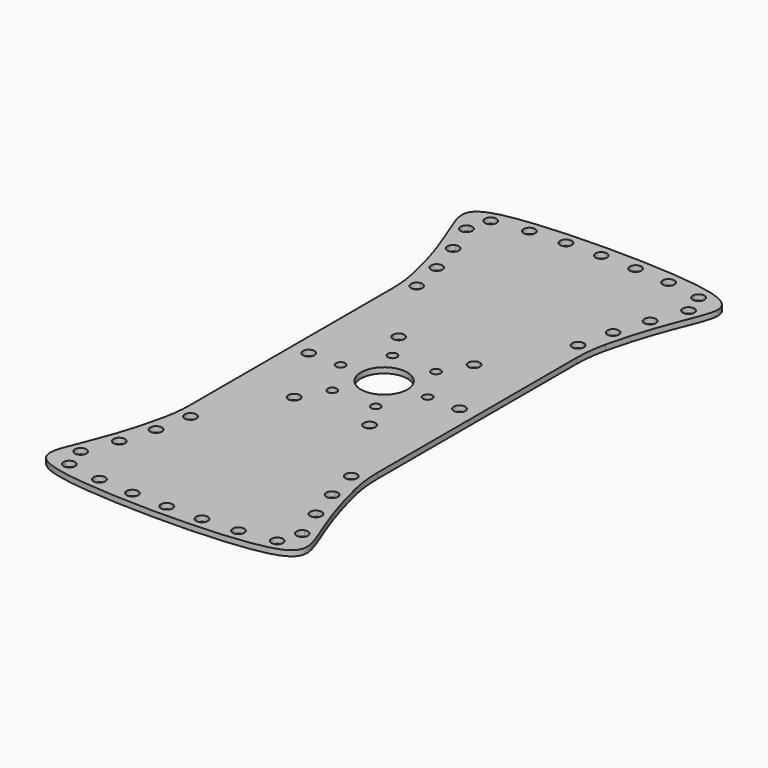
from build123d import *

# Parameters (mm, degrees)
F1_DEPTH = 2.9972
F2_R     = 2.54
F2_R_2   = 12.7
F3_DEPTH = 2.9982001
F4_R     = 3.175
F5_DEPTH = 2.9982001


# Not quite as in the source:
# - a feature names something its author has since deleted; it is built from what else it names


with BuildPart() as f1:
    # F0 (on Top) → F1 (new body)
    with BuildSketch(Plane.XY):
        with BuildLine():
            Line((-50.8, 69.1337430724), (-50.8, 0))
            ThreePointArc((-50.8, 0), (0, -50.8), (50.8, 0))
            Line((50.8, 0), (50.8, 68.084156834))
            ThreePointArc((50.8, 68.084156834), (51.3066265414, 76.856454963), (52.8197694085, 85.5121053476))
            add(Edge.make_bspline(
                [(-52.4169124656, 84.7479370585), (-59.7763542356, 119.901201468), (-79.0847149078, 143.3209937269), (-48.7989520232, 156.4254085379), (48.9543407971, 156.6289051226), (78.6905979985, 142.9845070095), (61.240777086, 121.355239199), (52.8197694085, 85.5121053476)],
                knots=[0.016652167, 0.016652167, 0.016652167, 0.016652167, 0.2315423779, 0.3598652356, 0.6401347644, 0.7684576221, 0.9823940037, 0.9823940037, 0.9823940037, 0.9823940037], degree=3))
            ThreePointArc((-52.4169124656, 84.7479370585), (-51.205306023, 76.982587888), (-50.8, 69.1337430724))
        make_face()
        with BuildLine():
            ThreePointArc((-40.8635060245, 77.3464568111), (-46.0941000823, 74.9267134219), (-44.5517945725, 80.47969154))
            ThreePointArc((-44.5517945725, 80.47969154), (-41.9829119668, 79.7662002004), (-40.8635060245, 77.3464568111))
        make_face(mode=Mode.SUBTRACT)
        with BuildLine():
            ThreePointArc((-44.8219086152, 95.9806605486), (-45.4423549678, 94.0952214319), (-47.0612035208, 92.9466729124))
            ThreePointArc((-47.0612035208, 92.9466729124), (-51.0712627717, 95.1875833011), (-48.645629391, 99.0886802324))
            ThreePointArc((-48.645629391, 99.0886802324), (-45.9942932581, 98.444429355), (-44.8219086152, 95.9806605486))
        make_face(mode=Mode.SUBTRACT)
        with BuildLine():
            ThreePointArc((-50.4062777497, 114.1937690523), (-50.9612142113, 112.4004782074), (-52.4320365242, 111.2340613632))
            ThreePointArc((-52.4320365242, 111.2340613632), (-56.5676237816, 113.1156399423), (-54.5876780098, 117.2050451135))
            ThreePointArc((-54.5876780098, 117.2050451135), (-51.7258392336, 116.7701954365), (-50.4062777497, 114.1937690523))
        make_face(mode=Mode.SUBTRACT)
        with BuildLine():
            ThreePointArc((-57.3376559554, 131.938021535), (-57.88209946, 130.1601583445), (-59.3287095139, 128.9920249594))
            ThreePointArc((-59.3287095139, 128.9920249594), (-63.4641851685, 130.7679359381), (-61.6688548547, 134.8950181711))
            ThreePointArc((-61.6688548547, 134.8950181711), (-58.7224473789, 134.5601920582), (-57.3376559554, 131.938021535))
        make_face(mode=Mode.SUBTRACT)
        with BuildLine():
            ThreePointArc((-53.7960603193, 144.1342135781), (-56.4975490613, 140.9947212483), (-60.0048238397, 143.1977821056))
            ThreePointArc((-60.0048238397, 143.1977821056), (-57.8198491671, 147.1936551107), (-53.8884721201, 144.8946575233))
            ThreePointArc((-53.8884721201, 144.8946575233), (-53.8192479413, 144.5172328122), (-53.7960603193, 144.1342135781))
        make_face(mode=Mode.SUBTRACT)
        with BuildLine():
            ThreePointArc((-34.9702627037, 147.0482904702), (-37.995578786, 143.8768208227), (-41.3061491445, 146.7492555085))
            ThreePointArc((-41.3061491445, 146.7492555085), (-38.4509946725, 150.2085361827), (-34.9856719085, 147.3607180735))
            ThreePointArc((-34.9856719085, 147.3607180735), (-34.9741173448, 147.2046941553), (-34.9702627037, 147.0482904702))
        make_face(mode=Mode.SUBTRACT)
        with BuildLine():
            ThreePointArc((-15.9590420103, 148.2631928317), (-19.0948463149, 145.0884347783), (-22.3080742607, 148.1848074146))
            ThreePointArc((-22.3080742607, 148.1848074146), (-19.2571889586, 151.4358037169), (-15.9634837046, 148.4310768101))
            ThreePointArc((-15.9634837046, 148.4310768101), (-15.9601526281, 148.3471641942), (-15.9590420103, 148.2631928317))
        make_face(mode=Mode.SUBTRACT)
        with BuildLine():
            ThreePointArc((47.2575965607, 77.582145781), (41.6326151645, 75.5626864082), (44.6886415002, 80.6987680763))
            ThreePointArc((44.6886415002, 80.6987680763), (46.5325779568, 79.6016051539), (47.2575965607, 77.582145781))
        make_face(mode=Mode.SUBTRACT)
        with BuildLine():
            ThreePointArc((47.4797824009, 93.1003405079), (45.3705359663, 96.9606098577), (49.1428743284, 99.2233655354))
            ThreePointArc((49.1428743284, 99.2233655354), (50.9174308294, 98.1072314537), (51.6095262724, 96.1283908938))
            ThreePointArc((51.6095262724, 96.1283908938), (50.3119331553, 93.5679283583), (47.4797824009, 93.1003405079))
        make_face(mode=Mode.SUBTRACT)
        with BuildLine():
            ThreePointArc((3.0909579897, 148.6372462056), (-0.1029362656, 145.4623024254), (-3.2588171329, 148.675034047))
            ThreePointArc((-3.2588171329, 148.675034047), (-0.0872347979, 151.8122446002), (3.0906506924, 148.6814190904))
            ThreePointArc((3.0906506924, 148.6814190904), (3.0908811644, 148.6593331824), (3.0909579897, 148.6372462056))
        make_face(mode=Mode.SUBTRACT)
        with BuildLine():
            ThreePointArc((22.137110859, 148.2255283412), (18.8449293043, 145.1249914855), (15.7921571233, 148.4615121573))
            ThreePointArc((15.7921571233, 148.4615121573), (19.044817873, 151.4717417271), (22.1379334659, 148.2977978171))
            ThreePointArc((22.1379334659, 148.2977978171), (22.1377278075, 148.2616607384), (22.137110859, 148.2255283412))
        make_face(mode=Mode.SUBTRACT)
        with BuildLine():
            ThreePointArc((41.1358520444, 146.797176727), (37.6674396013, 143.9372524612), (34.8157468695, 147.4124359448))
            ThreePointArc((34.8157468695, 147.4124359448), (38.132825935, 150.2683923102), (41.1500700749, 147.0973139308))
            ThreePointArc((41.1500700749, 147.0973139308), (41.1465135754, 146.9470770399), (41.1358520444, 146.797176727))
        make_face(mode=Mode.SUBTRACT)
        with BuildLine():
            ThreePointArc((52.9867605228, 111.3442691981), (51.1303654682, 115.3814686532), (55.1283946905, 117.3207840933))
            ThreePointArc((55.1283946905, 117.3207840933), (56.6965282926, 116.1646916046), (57.294259448, 114.3104234734))
            ThreePointArc((57.294259448, 114.3104234734), (55.9199455551, 111.6954369449), (52.9867605228, 111.3442691981))
        make_face(mode=Mode.SUBTRACT)
        with BuildLine():
            ThreePointArc((59.8190768743, 143.166925299), (55.922941879, 141.0690853743), (53.7138004196, 144.9032077333))
            ThreePointArc((53.7138004196, 144.9032077333), (57.1845775976, 147.2735561917), (59.9664431146, 144.1229895318))
            ThreePointArc((59.9664431146, 144.1229895318), (59.9293852896, 143.6393120499), (59.8190768743, 143.166925299))
        make_face(mode=Mode.SUBTRACT)
        with BuildLine():
            ThreePointArc((59.7670804201, 129.1468155623), (57.9403922201, 133.2339684449), (62.0166331459, 135.0848785944))
            ThreePointArc((62.0166331459, 135.0848785944), (63.5167589772, 133.9209947171), (64.0844760149, 132.109172277))
            ThreePointArc((64.0844760149, 132.109172277), (62.7057943311, 129.4911834484), (59.7670804201, 129.1468155623))
        make_face(mode=Mode.SUBTRACT)
    extrude(amount=F1_DEPTH)

    # F2 (on face) → F3 (cut, through all)
    with BuildSketch(Plane.XY.offset(2.9972)):
        with Locations((23.8125, 0)):
            Circle(F2_R)
        with Locations((11.90625, 20.6222299276)):
            Circle(F2_R)
        with Locations((-23.8125, 0)):
            Circle(F2_R)
        with Locations((-11.90625, -20.6222299276)):
            Circle(F2_R)
        with Locations((11.90625, -20.6222299276)):
            Circle(F2_R)
        with Locations((-11.90625, 20.6222299276)):
            Circle(F2_R)
        Circle(F2_R_2)
    extrude(amount=-F3_DEPTH, mode=Mode.SUBTRACT)

    # F4 (on face) → F5 (cut, through all)
    with BuildSketch(Plane.XY.offset(2.9972)):
        with Locations((-20.6375, 35.7451985412)):
            Circle(F4_R)
        with Locations((-41.275, 0)):
            Circle(F4_R)
        with Locations((-20.6375, -35.7451985412)):
            Circle(F4_R)
        with Locations((20.6375, -35.7451985412)):
            Circle(F4_R)
        with Locations((41.275, 0)):
            Circle(F4_R)
        with Locations((20.6375, 35.7451985412)):
            Circle(F4_R)
    extrude(amount=-F5_DEPTH, mode=Mode.SUBTRACT)

    # F6: F1 across plane


with BuildPart() as f1_1:
    add(f1.part)
    add(f1.part.mirror(Plane.XZ))


solid = f1_1.part
